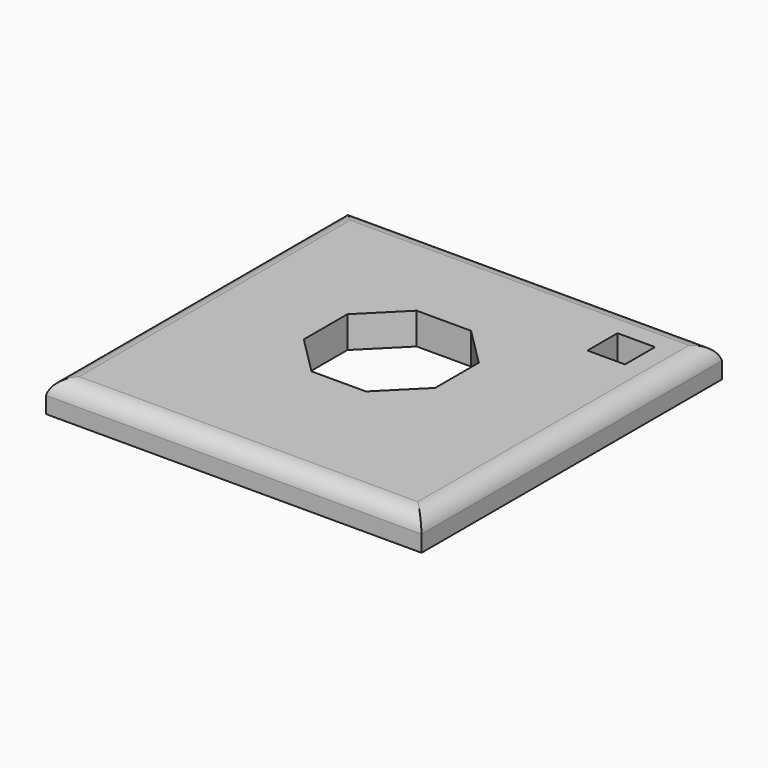
from build123d import *

# Parameters (mm, degrees)
F0_W        = 100
F0_H        = 100
F1_DEPTH    = 4
F3_T1_DEPTH = 124.4948974279
F3_T3_DEPTH = 124.4948974279
F5_DEPTH    = 25
F4_W        = 10
F4_H        = 10
F6_DEPTH    = 25
F7_DEPTH    = 4.4


# Not quite as in the source:
# - a fillet or chamfer that OpenCascade refuses, or shapes differently, is made with other operations: its cross-section is extruded or revolved along the edge and cut away or added


with BuildPart() as f1:
    # F0 (on Top) → F1 (new body)
    with BuildSketch(Plane.XY):
        with Locations((1.60311535, -4.4280775759)):
            Rectangle(F0_W, F0_H)
    extrude(amount=F1_DEPTH)

    # F3: fillet of radius 5 on 4 edges, made by hand

    # F3_s2 → F3_t1 (cut)
    with BuildSketch(Plane.YZ.offset(-60.6443333639)):
        with BuildLine():
            ThreePointArc((-54.4280775759, 0), (-52.6913757505, 2.8729833462), (-49.5290980903, 4))
            Line((-49.5290980903, 4), (-54.4280775759, 4))
            Line((-54.4280775759, 4), (-54.4280775759, 0))
        make_face()
        with BuildLine():
            ThreePointArc((45.5719224241, 0), (43.8352205987, 2.8729833462), (40.6729429385, 4))
            Line((40.6729429385, 4), (45.5719224241, 4))
            Line((45.5719224241, 4), (45.5719224241, 0))
        make_face()
    extrude(amount=F3_T1_DEPTH, mode=Mode.SUBTRACT)

    # F3_s4 → F3_t3 (cut)
    with BuildSketch(Plane.XZ.offset(-57.819371138)):
        with BuildLine():
            ThreePointArc((51.60311535, 0), (49.8664135246, 2.8729833462), (46.7041358644, 4))
            Line((46.7041358644, 4), (51.60311535, 4))
            Line((51.60311535, 4), (51.60311535, 0))
        make_face()
        with BuildLine():
            ThreePointArc((-48.39688465, 0), (-46.6601828246, 2.8729833462), (-43.4979051644, 4))
            Line((-43.4979051644, 4), (-48.39688465, 4))
            Line((-48.39688465, 4), (-48.39688465, 0))
        make_face()
    extrude(amount=F3_T3_DEPTH, mode=Mode.SUBTRACT)

    # F2 (on face) → F5 (cut)
    with BuildSketch(Plane.XY.offset(4)):
        Polygon((-7.2487373415, -17.5), (7.2487373415, -17.5), (17.5, -7.2487373415), (17.5, 7.2487373415), (7.2487373415, 17.5), (-7.2487373415, 17.5), (-17.5, 7.2487373415), (-17.5, -7.2487373415), align=None)
    extrude(amount=-F5_DEPTH, mode=Mode.SUBTRACT)

    # F4 (on face) → F6 (cut)
    with BuildSketch(Plane.XY.offset(4)):
        with Locations((36.7041358644, 30.6729429385)):
            Rectangle(F4_W, F4_H)
    extrude(amount=-F6_DEPTH, mode=Mode.SUBTRACT)

    # F7 (add): a face of the model
    f7_faces = [f1.faces().sort_by_distance(p)[0] for p in [
        (1.60311535, -53.0138640135, 0),
    ]]
    extrude(f7_faces, amount=F7_DEPTH)


solid = f1.part
